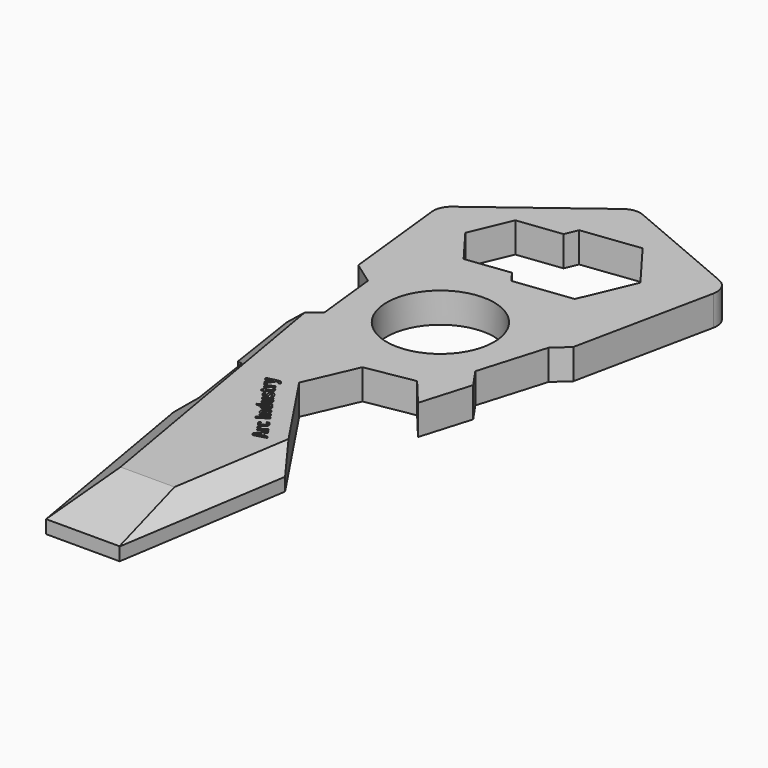
from build123d import *

# Parameters (mm, degrees)
F2_DEPTH      = 5
F3_R          = 8.8910509955
F4_DEPTH      = 5
F6_DEPTH      = 5
F8_DEPTH      = 5
F9_DEPTH      = 5
F11_SIZE2     = 2.8008301528
F11_SIZE      = 4
F12_SIZE2     = 2.805746614
F12_SIZE      = 13.2
F13_SIZE2     = 2.8342441162
F13_SIZE      = 3.5
F15_DEPTH     = 2
F16_R         = 3
F17_R         = 3
F18_TEXT_SIZE = 2.7351802504
F19_DEPTH     = 0.5
F20_R         = 3
F21_R         = 5
F22_DEPTH     = 25
F23_R         = 1


# Not quite as in the source:
# - Text() gives the source's letters only with a copy of the font that has no kerning and outlines rounded to 1/6400 em; it was checked with that copy


with BuildPart() as f2:
    # F1 (on face) → F2 (new body)
    with BuildSketch(Plane.XY):
        Polygon((17.7674815059, 33.2440920174), (23.069228977, 58.6924813688), (0, 68.5007199645), (-20.4051043838, 53.1256459653), (-18.284406513, 33.7742678821), (-14.5731819794, 31.1233922839), (-13.4253388629, 20.6493184276), (-17.2240566462, 17.6039338112), (-15.9452675514, 5.9349772838), (-13.4253388629, 3.5543027334), (-12.3040941173, -6.6770608635), (-14.5731819794, -9.169892408), (-8.7412586436, -42.8359918296), (3.4527601674, -42.8359918296), (7.9592475668, -14.2065538093), (-3.7045993377, 3.2892152667), (0, 11.772012338), (7.9592475668, 13.1507797752), (11.8435691245, 8.4743370716), (14.3213439733, 16.8086718768), (11.4053832367, 17.6755789956), (12.1039015062, 20.0251407924), (15.3879209983, 31.0713897959), align=None)
    extrude(amount=F2_DEPTH)

    # F3 (on face) → F4 (cut)
    with BuildSketch(Plane.XY.offset(5)):
        with Locations((0, 27.9197320342)):
            Circle(F3_R)
    extrude(amount=-F4_DEPTH, mode=Mode.SUBTRACT)

    # F5 (on face) → F6 (cut)
    with BuildSketch(Plane.XY.offset(5)):
        Polygon((9.5134102112, 43.8676981138), (13.2859320248, 52.7407662688), (7.4878904999, 60.4444000732), (-2.0826728387, 59.2749657227), (-5.8551946523, 50.4018975677), (-0.0571531274, 42.6982637632), align=None)
    extrude(amount=-F6_DEPTH, mode=Mode.SUBTRACT)

    # F7 (on face) → F8 (cut)
    with BuildSketch(Plane.XY.offset(5)):
        Polygon((-8.7297365832, 43.6409011503), (-1.4372709654, 44.5319730227), (-5.8551946523, 50.4018975677), (-2.9806527215, 57.1628939851), (-10.2731183393, 56.2718221128), (-13.1476602701, 49.5108256954), align=None)
    extrude(amount=-F8_DEPTH, mode=Mode.SUBTRACT)

    # F0 (on Top) → F9 (join)
    with BuildSketch(Plane.XY):
        Polygon((14.3213439733, 16.8086718768), (12.1039015062, 20.0251407924), (11.4053832367, 17.6755789956), align=None)
    extrude(amount=F9_DEPTH)

    # F11
    f11_edges = [f2.edges().sort_by_distance(p)[0] for p in [
        (-11.65722, -26.002942, 5),
    ]]
    f11_side = f2.faces().sort_by_distance((-1.393238, 15.763428, 5))[0]
    chamfer(f11_edges, length=F11_SIZE, length2=F11_SIZE2, reference=f11_side)

    # F12
    f12_edges = [f2.edges().sort_by_distance(p)[0] for p in [
        (-0.614463, -42.835992, 5),
    ]]
    f12_side = f2.faces().sort_by_distance((-13.667209, 18.923505, 5))[0]
    chamfer(f12_edges, length=F12_SIZE, length2=F12_SIZE2, reference=f12_side)

    # F13
    f13_edges = [f2.edges().sort_by_distance(p)[0] for p in [
        (6.744893, -21.921273, 5),
    ]]
    f13_side = f2.faces().sort_by_distance((-10.128706, -5.10339, 5))[0]
    chamfer(f13_edges, length=F13_SIZE, length2=F13_SIZE2, reference=f13_side)

    # F16
    f16_edges = [f2.edges().sort_by_distance(p)[0] for p in [
        (23.069229, 58.692481, 2.5),
    ]]
    fillet(f16_edges, radius=F16_R)

    # F17
    f17_edges = [f2.edges().sort_by_distance(p)[0] for p in [
        (-20.405104, 53.125646, 2.5),
    ]]
    fillet(f17_edges, radius=F17_R)

    # F18 (on face) → F19 (cut)
    with BuildSketch(Plane.XY.offset(5)):
        with Locations(Location((2.7726959439, -11.4137201791), (0, 0, 124.401581412))):
            Text('Arc Industry', F18_TEXT_SIZE, font='Open Sans', font_style=FontStyle.BOLD, text_align=(TextAlign.LEFT, TextAlign.BOTTOM))
    extrude(amount=-F19_DEPTH, mode=Mode.SUBTRACT)

    # F20
    f20_edges = [f2.edges().sort_by_distance(p)[0] for p in [
        (0, 68.50072, 2.5),
    ]]
    fillet(f20_edges, radius=F20_R)

    # F0 (on Top) → F22 (cut)
    with BuildSketch(Plane.XY):
        Polygon((11.4053832367, 7.000438869), (11.8435691245, 8.4743370716), (7.9592475668, 13.1507797752), align=None)
    extrude(amount=F22_DEPTH, mode=Mode.SUBTRACT)


with BuildPart() as f15:
    # F14 (on Top) → F15 (new body)
    with BuildSketch(Plane.XY):
        Polygon((-9.4787562266, 64.1314014792), (-9.4787562266, 61.5306347609), (0, 68.5448125005), (11.0909026116, 63.8949647546), (11.0909026116, 66.6533485055), (0, 71.3031962514), align=None)
    extrude(amount=F15_DEPTH)

    # F21
    f21_edges = [f15.edges().sort_by_distance(p)[0] for p in [
        (0, 68.544813, 1),
    ]]
    fillet(f21_edges, radius=F21_R)

    # F23
    f23_edges = [f15.edges().sort_by_distance(p)[0] for p in [
        (0, 71.303196, 1),
    ]]
    fillet(f23_edges, radius=F23_R)


solid = Compound([f2.part, f15.part])
